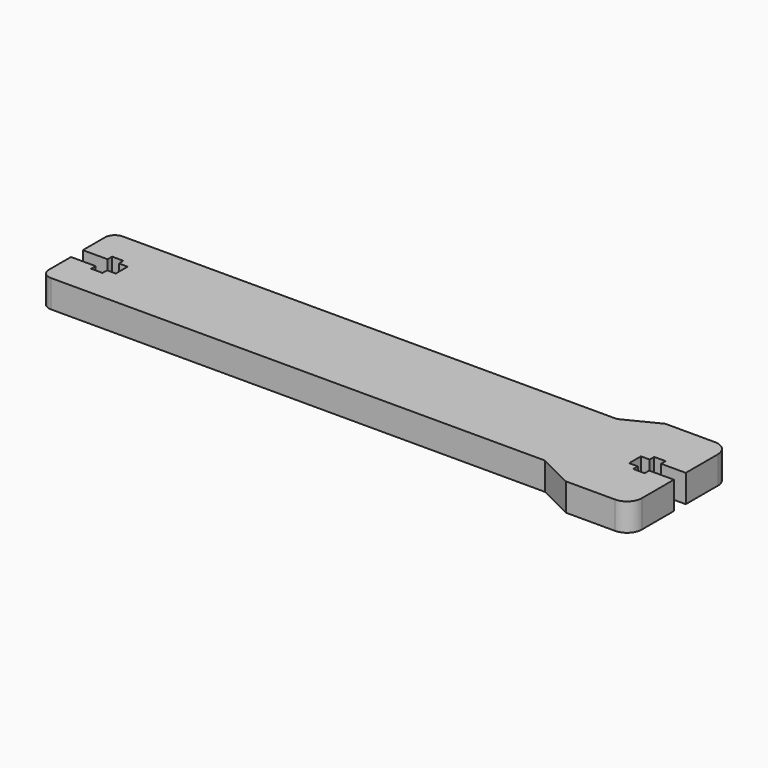
from build123d import *

# Parameters (mm, degrees)
F1_DEPTH = 5.588
F2_W     = 20
F2_H     = 5.588
F3_DEPTH = 3.5
F4_SIZE2 = 6.99999
F4_SIZE  = 3.49999
F5_W     = 20
F5_H     = 5.588
F6_DEPTH = 3.5
F7_SIZE2 = 3.49999
F7_SIZE  = 6.99999
F8_R     = 3


# Not quite as in the source:
# - a fillet or chamfer is up to 0.001 mm smaller than in the source, because OpenCascade refuses the exact size


with BuildPart() as f1:
    # F0 (on Top) → F1 (new body)
    with BuildSketch(Plane.XY):
        with BuildLine():
            Line((61, 9.1), (-59, 9.1))
            ThreePointArc((-59, 9.1), (-60.4142135624, 8.5142135624), (-61, 7.1))
            Line((-61, 7.1), (-61, 1.5))
            Line((-61, 1.5), (-56, 1.5))
            Line((-56, 1.5), (-56, 2.65))
            Line((-56, 2.65), (-53.7, 2.65))
            Line((-53.7, 2.65), (-53.7, 1.5))
            Line((-53.7, 1.5), (-51.934869796, 1.5))
            Line((-51.934869796, 1.5), (-51.934869796, -1.5))
            Line((-51.934869796, -1.5), (-53.7, -1.5))
            Line((-53.7, -1.5), (-53.7, -2.65))
            Line((-53.7, -2.65), (-56, -2.65))
            Line((-56, -2.65), (-56, -1.5))
            Line((-56, -1.5), (-61, -1.5))
            Line((-61, -1.5), (-61, -7.1))
            ThreePointArc((-61, -7.1), (-60.4142135624, -8.5142135624), (-59, -9.1))
            Line((-59, -9.1), (61, -9.1))
            Line((61, -9.1), (61, -7.1))
            Line((61, -7.1), (61, -1.5))
            Line((61, -1.5), (56, -1.5))
            Line((56, -1.5), (56, -2.65))
            Line((56, -2.65), (53.7, -2.65))
            Line((53.7, -2.65), (53.7, -1.5))
            Line((53.7, -1.5), (51.934869796, -1.5))
            Line((51.934869796, -1.5), (51.934869796, 1.5))
            Line((51.934869796, 1.5), (53.7, 1.5))
            Line((53.7, 1.5), (53.7, 2.65))
            Line((53.7, 2.65), (56, 2.65))
            Line((56, 2.65), (56, 1.5))
            Line((56, 1.5), (61, 1.5))
            Line((61, 1.5), (61, 7.1))
            Line((61, 7.1), (61, 9.1))
        make_face()
    extrude(amount=F1_DEPTH)

    # F2 (on face) → F3 (join)
    with BuildSketch(Plane(origin=(0, 9.1, 0), x_dir=(-1, 0, 0), z_dir=(0, 1, 0))):
        with Locations((-51, 2.794)):
            Rectangle(F2_W, F2_H)
    extrude(amount=F3_DEPTH)

    # F4 (size 3.5 and 7 in the source; OpenCascade refuses exactly that, so slightly less here)
    f4_edges = [f1.edges().sort_by_distance(p)[0] for p in [
        (41, 12.6, 2.794),
    ]]
    f4_side = f1.faces().sort_by_distance((41, 10.85, 2.794))[0]
    chamfer(f4_edges, length=F4_SIZE, length2=F4_SIZE2, reference=f4_side)

    # F5 (on face) → F6 (join)
    with BuildSketch(Plane.XZ.offset(9.1)):
        with Locations((51, 2.794)):
            Rectangle(F5_W, F5_H)
    extrude(amount=F6_DEPTH)

    # F7 (size 7 and 3.5 in the source; OpenCascade refuses exactly that, so slightly less here)
    f7_edges = [f1.edges().sort_by_distance(p)[0] for p in [
        (41, -12.6, 2.794),
    ]]
    f7_side = f1.faces().sort_by_distance((51, -12.6, 2.794))[0]
    chamfer(f7_edges, length=F7_SIZE, length2=F7_SIZE2, reference=f7_side)

    # F8
    f8_edges = [f1.edges().sort_by_distance(p)[0] for p in [
        (61, 12.6, 2.794),
        (61, -12.6, 2.794),
    ]]
    fillet(f8_edges, radius=F8_R)


solid = f1.part
